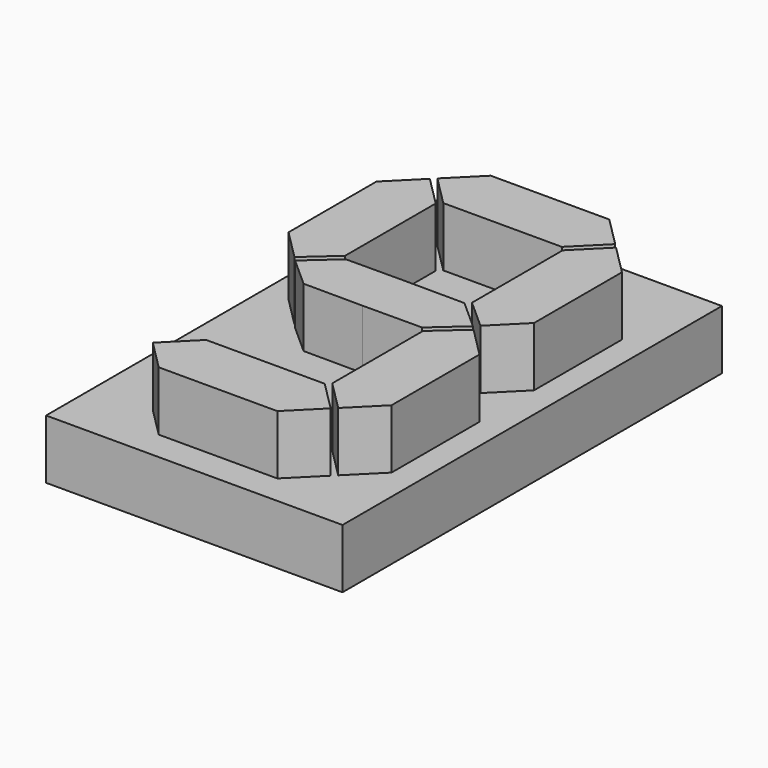
from build123d import *

# Parameters (mm, degrees)
F0_W     = 10
F0_H     = 16
F1_DEPTH = 2
F3_DEPTH = 2


# Not quite as in the source:
# - ends of sketch curves that miss each other by under 0.0002 mm in the source are joined


with BuildPart() as f1:
    # F0 (on Top) → F1 (new body)
    with BuildSketch(Plane.XY):
        Rectangle(F0_W, F0_H)
    extrude(amount=F1_DEPTH)

    # F2 (on face) → F3 (join)
    with BuildSketch(Plane.XY.offset(2)):
        Polygon((0, 7), (-2, 7), (-3, 6), (-2, 5), (0, 5), (2, 5), (3, 6), (2, 7), align=None)
        Polygon((-2.1414213562, 4.8585786438), (-3.1414213562, 5.8585786438), (-4.1414213562, 4.8585786438), (-4.1414213562, 1.1507223826), (-3.1374518146, 0.1453992321), (-2.1414213562, 1.0335195075), align=None)
        Polygon((2, 0.891659756), (2.00782e-05, 0.9006214721), (-2, 0.891659756), (-3, 0), (-2, -0.891659756), (-2.00782e-05, -0.9006214721), (2, -0.891659756), (3, 0), align=None)
        Polygon((0, -5), (-2, -5), (-3, -6), (-2, -7), (0, -7), (2, -7), (3, -6), (2, -5), align=None)
        Polygon((4.1414213562, 4.8585786438), (3.1414213562, 5.8585786438), (2.1414213562, 4.8585786438), (2.1414213562, 1.0335195075), (3.1374518146, 0.1453992321), (4.1414213562, 1.1507223826), align=None)
        Polygon((3.1374518146, -0.1453992321), (2.1414213562, -1.0335195075), (2.1414213562, -4.8585786438), (3.1414213562, -5.8585786438), (4.1414213562, -4.8585786438), (4.1414213562, -1.1507223826), align=None)
    extrude(amount=F3_DEPTH)


solid = f1.part
